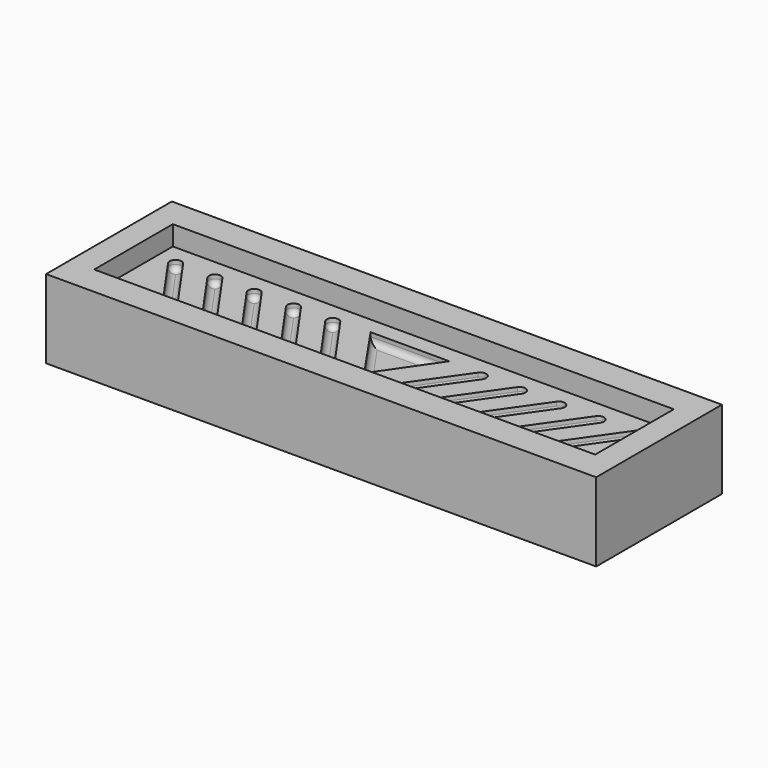
from build123d import *

# Parameters (mm, degrees)
F0_W     = 35.56
F0_H     = 10.16
F1_DEPTH = 5.08
F2_W     = 32.385
F2_H     = 6.35
F3_DEPTH = 1.27
F5_DEPTH = 0.635
F6_R     = 0.38099


# Not quite as in the source:
# - a fillet or chamfer is up to 0.001 mm smaller than in the source, because OpenCascade refuses the exact size


with BuildPart() as f1:
    # F0 (on Top) → F1 (new body)
    with BuildSketch(Plane.XY):
        Rectangle(F0_W, F0_H)
    extrude(amount=F1_DEPTH)

    # F2 (on face) → F3 (cut)
    with BuildSketch(Plane.XY.offset(5.08)):
        Rectangle(F2_W, F2_H)
    extrude(amount=-F3_DEPTH, mode=Mode.SUBTRACT)

    # F4 (on face) → F5 (cut)
    with BuildSketch(Plane.XY.offset(3.81)):
        with BuildLine():
            ThreePointArc((-14.6151767009, 2.0390980407), (-15.145806252, 2.1326623473), (-15.2393705587, 1.6020327962))
            Line((-15.2393705587, 1.6020327962), (-12.6898232991, -2.0390980407))
            ThreePointArc((-12.6898232991, -2.0390980407), (-12.159193748, -2.1326623473), (-12.0656294413, -1.6020327962))
            Line((-12.0656294413, -1.6020327962), (-14.6151767009, 2.0390980407))
        make_face()
        with BuildLine():
            Line((-9.5256294413, -1.6020327962), (-12.0751767009, 2.0390980407))
            ThreePointArc((-12.0751767009, 2.0390980407), (-12.605806252, 2.1326623473), (-12.6993705587, 1.6020327962))
            Line((-12.6993705587, 1.6020327962), (-10.1498232991, -2.0390980407))
            ThreePointArc((-10.1498232991, -2.0390980407), (-9.619193748, -2.1326623473), (-9.5256294413, -1.6020327962))
        make_face()
        with BuildLine():
            Line((-6.9856294413, -1.6020327962), (-9.5351767009, 2.0390980407))
            ThreePointArc((-9.5351767009, 2.0390980407), (-10.065806252, 2.1326623473), (-10.1593705587, 1.6020327962))
            Line((-10.1593705587, 1.6020327962), (-7.6098232991, -2.0390980407))
            ThreePointArc((-7.6098232991, -2.0390980407), (-7.079193748, -2.1326623473), (-6.9856294413, -1.6020327962))
        make_face()
        with BuildLine():
            Line((-4.4456294413, -1.6020327962), (-6.9951767009, 2.0390980407))
            ThreePointArc((-6.9951767009, 2.0390980407), (-7.525806252, 2.1326623473), (-7.6193705587, 1.6020327962))
            Line((-7.6193705587, 1.6020327962), (-5.0698232991, -2.0390980407))
            ThreePointArc((-5.0698232991, -2.0390980407), (-4.539193748, -2.1326623473), (-4.4456294413, -1.6020327962))
        make_face()
        with BuildLine():
            Line((-1.9056294413, -1.6020327962), (-4.4551767009, 2.0390980407))
            ThreePointArc((-4.4551767009, 2.0390980407), (-4.985806252, 2.1326623473), (-5.0793705587, 1.6020327962))
            Line((-5.0793705587, 1.6020327962), (-2.5298232991, -2.0390980407))
            ThreePointArc((-2.5298232991, -2.0390980407), (-1.999193748, -2.1326623473), (-1.9056294413, -1.6020327962))
        make_face()
        with BuildLine():
            Line((12.6898232991, -2.0390980407), (15.2393705587, 1.6020327962))
            ThreePointArc((15.2393705587, 1.6020327962), (15.145806252, 2.1326623473), (14.6151767009, 2.0390980407))
            Line((14.6151767009, 2.0390980407), (12.0656294413, -1.6020327962))
            ThreePointArc((12.0656294413, -1.6020327962), (12.159193748, -2.1326623473), (12.6898232991, -2.0390980407))
        make_face()
        with BuildLine():
            Line((10.1498232991, -2.0390980407), (12.6993705587, 1.6020327962))
            ThreePointArc((12.6993705587, 1.6020327962), (12.605806252, 2.1326623473), (12.0751767009, 2.0390980407))
            Line((12.0751767009, 2.0390980407), (9.5256294413, -1.6020327962))
            ThreePointArc((9.5256294413, -1.6020327962), (9.619193748, -2.1326623473), (10.1498232991, -2.0390980407))
        make_face()
        with BuildLine():
            Line((9.5351767009, 2.0390980407), (6.9856294413, -1.6020327962))
            ThreePointArc((6.9856294413, -1.6020327962), (7.079193748, -2.1326623473), (7.6098232991, -2.0390980407))
            Line((7.6098232991, -2.0390980407), (10.1593705587, 1.6020327962))
            ThreePointArc((10.1593705587, 1.6020327962), (10.065806252, 2.1326623473), (9.5351767009, 2.0390980407))
        make_face()
        with BuildLine():
            Line((5.0698232991, -2.0390980407), (7.6193705587, 1.6020327962))
            ThreePointArc((7.6193705587, 1.6020327962), (7.525806252, 2.1326623473), (6.9951767009, 2.0390980407))
            Line((6.9951767009, 2.0390980407), (4.4456294413, -1.6020327962))
            ThreePointArc((4.4456294413, -1.6020327962), (4.539193748, -2.1326623473), (5.0698232991, -2.0390980407))
        make_face()
        with BuildLine():
            Line((2.5298232991, -2.0390980407), (5.0793705587, 1.6020327962))
            ThreePointArc((5.0793705587, 1.6020327962), (4.985806252, 2.1326623473), (4.4551767009, 2.0390980407))
            Line((4.4551767009, 2.0390980407), (1.9056294413, -1.6020327962))
            ThreePointArc((1.9056294413, -1.6020327962), (1.999193748, -2.1326623473), (2.5298232991, -2.0390980407))
        make_face()
        Polygon((-2.5421355385, 2.0958390087), (0, -1.6020327962), (0, 2.0958390087), align=None)
        Polygon((0, 2.0958390087), (0, -1.6020327962), (2.5421355385, 2.0958390087), align=None)
    extrude(amount=-F5_DEPTH, mode=Mode.SUBTRACT)

    # F6 (radius 0.381 in the source; OpenCascade refuses exactly that, so slightly less here)
    f6_edges = [f1.edges().sort_by_distance(p)[0] for p in [
        (-10.800403, 0.218533, 3.175),
        (-13.964597, -0.218533, 3.175),
        (-8.884597, -0.218533, 3.175),
        (-6.344597, -0.218533, 3.175),
        (-3.804597, -0.218533, 3.175),
        (3.180403, 0.218533, 3.175),
        (5.720403, 0.218533, 3.175),
        (8.260403, 0.218533, 3.175),
        (10.800403, 0.218533, 3.175),
        (13.340403, 0.218533, 3.175),
        (0, 2.095839, 3.175),
        (-1.271068, 0.246903, 3.175),
        (1.271068, 0.246903, 3.175),
    ]]
    fillet(f6_edges, radius=F6_R)


solid = f1.part
